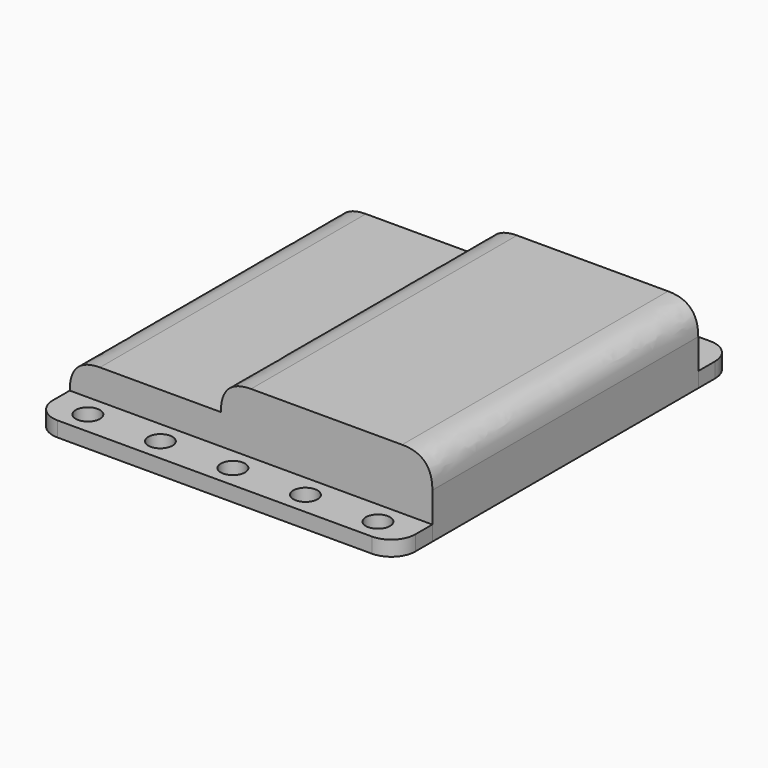
from build123d import *

# Parameters (mm, degrees)
F1_DEPTH    = 3.175
F0_W        = 76.2
F0_H        = 69.85
F2_DEPTH    = 9.525
F3_W        = 44.45
F3_H        = 69.85
F4_DEPTH    = 6.35
F5_T1_DEPTH = 101.6
F6_R        = 5.08
F6_2_R      = 5.08


# Not quite as in the source:
# - a fillet or chamfer that OpenCascade refuses, or shapes differently, is made with other operations: its cross-section is extruded or revolved along the edge and cut away or added


with BuildPart() as f1:
    # F0 (on Top) → F1 (new body)
    with BuildSketch(Plane.XY):
        with BuildLine():
            Line((-45.1224932384, -53.3683788409), (-50.2024932384, -53.3683788409))
            Line((-50.2024932384, -53.3683788409), (-50.2024932384, -58.1308788409))
            Line((-50.2024932384, -58.1308788409), (25.9975067616, -58.1308788409))
            Line((25.9975067616, -58.1308788409), (25.9975067616, -53.3683788409))
            Line((25.9975067616, -53.3683788409), (20.9175067616, -53.3683788409))
            ThreePointArc((20.9175067616, -53.3683788409), (18.3775067616, -55.9083788409), (15.8375067616, -53.3683788409))
            Line((15.8375067616, -53.3683788409), (5.6775067616, -53.3683788409))
            ThreePointArc((5.6775067616, -53.3683788409), (3.1375067616, -55.9083788409), (0.5975067616, -53.3683788409))
            Line((0.5975067616, -53.3683788409), (-9.5624932384, -53.3683788409))
            ThreePointArc((-9.5624932384, -53.3683788409), (-12.1024932384, -55.9083788409), (-14.6424932384, -53.3683788409))
            Line((-14.6424932384, -53.3683788409), (-24.8024932384, -53.3683788409))
            ThreePointArc((-24.8024932384, -53.3683788409), (-27.3424932384, -55.9083788409), (-29.8824932384, -53.3683788409))
            Line((-29.8824932384, -53.3683788409), (-40.0424932384, -53.3683788409))
            ThreePointArc((-40.0424932384, -53.3683788409), (-42.5824932384, -55.9083788409), (-45.1224932384, -53.3683788409))
        make_face()
        with BuildLine():
            Line((25.9975067616, -48.6058788409), (-50.2024932384, -48.6058788409))
            Line((-50.2024932384, -48.6058788409), (-50.2024932384, -53.3683788409))
            Line((-50.2024932384, -53.3683788409), (-45.1224932384, -53.3683788409))
            ThreePointArc((-45.1224932384, -53.3683788409), (-42.5824932384, -50.8283788409), (-40.0424932384, -53.3683788409))
            Line((-40.0424932384, -53.3683788409), (-29.8824932384, -53.3683788409))
            ThreePointArc((-29.8824932384, -53.3683788409), (-27.3424932384, -50.8283788409), (-24.8024932384, -53.3683788409))
            Line((-24.8024932384, -53.3683788409), (-14.6424932384, -53.3683788409))
            ThreePointArc((-14.6424932384, -53.3683788409), (-12.1024932384, -50.8283788409), (-9.5624932384, -53.3683788409))
            Line((-9.5624932384, -53.3683788409), (0.5975067616, -53.3683788409))
            ThreePointArc((0.5975067616, -53.3683788409), (3.1375067616, -50.8283788409), (5.6775067616, -53.3683788409))
            Line((5.6775067616, -53.3683788409), (15.8375067616, -53.3683788409))
            ThreePointArc((15.8375067616, -53.3683788409), (18.3775067616, -50.8283788409), (20.9175067616, -53.3683788409))
            Line((20.9175067616, -53.3683788409), (25.9975067616, -53.3683788409))
            Line((25.9975067616, -53.3683788409), (25.9975067616, -48.6058788409))
        make_face()
    extrude(amount=F1_DEPTH)

    # F6#2
    f6_2_edges = [f1.edges().sort_by_distance(p)[0] for p in [
        (-50.202493, -58.130879, 1.5875),
        (25.997507, -58.130879, 1.5875),
    ]]
    fillet(f6_2_edges, radius=F6_2_R)


with BuildPart() as f1b:
    # F0 (on Top) → F1, piece 2 (new body)
    with BuildSketch(Plane.XY):
        with BuildLine():
            Line((-45.1224932384, 26.0066211591), (-50.2024932384, 26.0066211591))
            Line((-50.2024932384, 26.0066211591), (-50.2024932384, 21.2441211591))
            Line((-50.2024932384, 21.2441211591), (25.9975067616, 21.2441211591))
            Line((25.9975067616, 21.2441211591), (25.9975067616, 26.0066211591))
            Line((25.9975067616, 26.0066211591), (20.9175067616, 26.0066211591))
            ThreePointArc((20.9175067616, 26.0066211591), (18.3775067616, 23.4666211591), (15.8375067616, 26.0066211591))
            Line((15.8375067616, 26.0066211591), (5.6775067616, 26.0066211591))
            ThreePointArc((5.6775067616, 26.0066211591), (3.1375067616, 23.4666211591), (0.5975067616, 26.0066211591))
            Line((0.5975067616, 26.0066211591), (-9.5624932384, 26.0066211591))
            ThreePointArc((-9.5624932384, 26.0066211591), (-12.1024932384, 23.4666211591), (-14.6424932384, 26.0066211591))
            Line((-14.6424932384, 26.0066211591), (-24.8024932384, 26.0066211591))
            ThreePointArc((-24.8024932384, 26.0066211591), (-27.3424932384, 23.4666211591), (-29.8824932384, 26.0066211591))
            Line((-29.8824932384, 26.0066211591), (-40.0424932384, 26.0066211591))
            ThreePointArc((-40.0424932384, 26.0066211591), (-42.5824932384, 23.4666211591), (-45.1224932384, 26.0066211591))
        make_face()
        with BuildLine():
            Line((25.9975067616, 30.7691211591), (-50.2024932384, 30.7691211591))
            Line((-50.2024932384, 30.7691211591), (-50.2024932384, 26.0066211591))
            Line((-50.2024932384, 26.0066211591), (-45.1224932384, 26.0066211591))
            ThreePointArc((-45.1224932384, 26.0066211591), (-42.5824932384, 28.5466211591), (-40.0424932384, 26.0066211591))
            Line((-40.0424932384, 26.0066211591), (-29.8824932384, 26.0066211591))
            ThreePointArc((-29.8824932384, 26.0066211591), (-27.3424932384, 28.5466211591), (-24.8024932384, 26.0066211591))
            Line((-24.8024932384, 26.0066211591), (-14.6424932384, 26.0066211591))
            ThreePointArc((-14.6424932384, 26.0066211591), (-12.1024932384, 28.5466211591), (-9.5624932384, 26.0066211591))
            Line((-9.5624932384, 26.0066211591), (0.5975067616, 26.0066211591))
            ThreePointArc((0.5975067616, 26.0066211591), (3.1375067616, 28.5466211591), (5.6775067616, 26.0066211591))
            Line((5.6775067616, 26.0066211591), (15.8375067616, 26.0066211591))
            ThreePointArc((15.8375067616, 26.0066211591), (18.3775067616, 28.5466211591), (20.9175067616, 26.0066211591))
            Line((20.9175067616, 26.0066211591), (25.9975067616, 26.0066211591))
            Line((25.9975067616, 26.0066211591), (25.9975067616, 30.7691211591))
        make_face()
    extrude(amount=F1_DEPTH)

    # F6
    f6_edges = [f1b.edges().sort_by_distance(p)[0] for p in [
        (25.997507, 30.769121, 1.5875),
        (-50.202493, 30.769121, 1.5875),
    ]]
    fillet(f6_edges, radius=F6_R)


with BuildPart() as f2:
    # F0 (on Top) → F2 (new body)
    with BuildSketch(Plane.XY):
        with Locations((-12.1024932384, -13.6808788409)):
            Rectangle(F0_W, F0_H)
    extrude(amount=F2_DEPTH)

    # F3 (on face) → F4 (join)
    with BuildSketch(Plane.XY.offset(9.525)):
        with Locations((3.7725067616, -13.6808788409)):
            Rectangle(F3_W, F3_H)
    extrude(amount=F4_DEPTH)

    # F5: fillet of radius 6.35 on 3 edges, made by hand

    # F5_s2 → F5_t1 (cut)
    with BuildSketch(Plane.XZ.offset(-37.1191211591)):
        with BuildLine():
            add(Edge.make_bspline(
                [(-18.4524932384, 9.525), (-18.4524932384, 15.875), (-12.1024932384, 15.875)],
                knots=[0, 0, 0, 1, 1, 1], degree=2, weights=[1, 1, 1]))
            Line((-12.1024932384, 15.875), (-18.4524932384, 15.875))
            Line((-18.4524932384, 15.875), (-18.4524932384, 9.525))
        make_face()
        with BuildLine():
            add(Edge.make_bspline(
                [(25.9975067616, 9.525), (25.9975067616, 15.875), (19.6475067616, 15.875)],
                knots=[0, 0, 0, 1, 1, 1], degree=2, weights=[1, 1, 1]))
            Line((19.6475067616, 15.875), (25.9975067616, 15.875))
            Line((25.9975067616, 15.875), (25.9975067616, 9.525))
        make_face()
        with BuildLine():
            add(Edge.make_bspline(
                [(-50.2024932384, 3.175), (-50.2024932384, 9.525), (-43.8524932384, 9.525)],
                knots=[0, 0, 0, 1, 1, 1], degree=2, weights=[1, 1, 1]))
            Line((-43.8524932384, 9.525), (-50.2024932384, 9.525))
            Line((-50.2024932384, 9.525), (-50.2024932384, 3.175))
        make_face()
    extrude(amount=F5_T1_DEPTH, mode=Mode.SUBTRACT)


solid = Compound([f1.part, f1b.part, f2.part])
